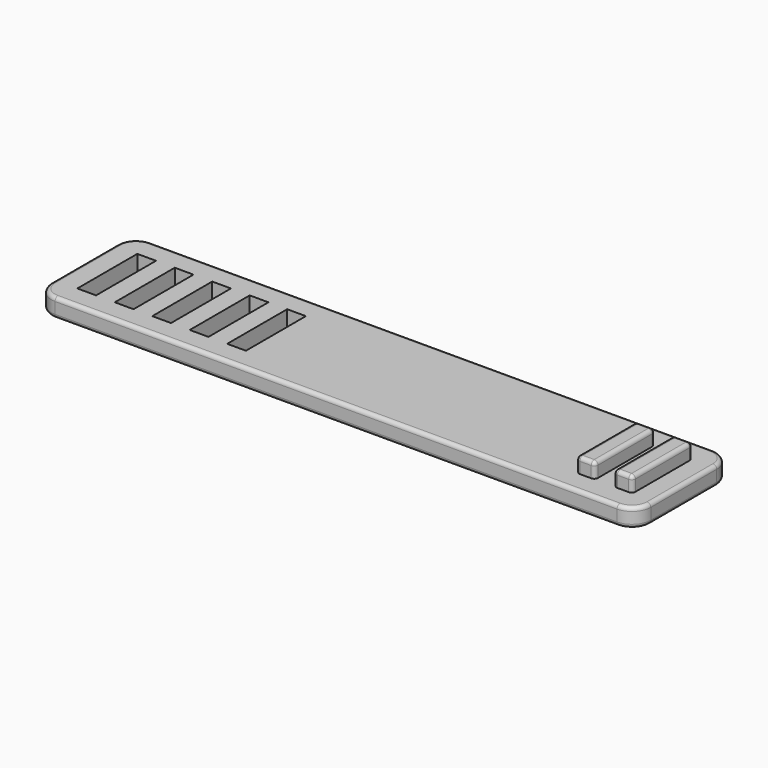
from build123d import *

# Parameters (mm, degrees)
F0_W     = 6.35
F0_H     = 25.4
F0_R     = 17.5576306553
F1_DEPTH = 6.35
F2_R     = 1.27
F3_W     = 6.35
F3_H     = 25.4
F4_DEPTH = 5.08
F5_R     = 1.27


# Not quite as in the source:
# - a feature names something its author has since deleted; it is built from what else it names


with BuildPart() as f1:
    # F0 (on Top) → F1 (new body)
    with BuildSketch(Plane.XY):
        with BuildLine():
            ThreePointArc((101.6, 13.97), (99.7401280605, 18.4601280605), (95.25, 20.32))
            Line((95.25, 20.32), (-95.25, 20.32))
            ThreePointArc((-95.25, 20.32), (-99.7401280605, 18.4601280605), (-101.6, 13.97))
            Line((-101.6, 13.97), (-101.6, -13.97))
            ThreePointArc((-101.6, -13.97), (-99.7401280605, -18.4601280605), (-95.25, -20.32))
            Line((-95.25, -20.32), (95.25, -20.32))
            ThreePointArc((95.25, -20.32), (99.7401280605, -18.4601280605), (101.6, -13.97))
            Line((101.6, -13.97), (101.6, 13.97))
        make_face()
        with Locations((-90.6151607633, 0)):
            Rectangle(F0_W, F0_H, mode=Mode.SUBTRACT)
        with Locations((-77.9151607633, 0)):
            Rectangle(F0_W, F0_H, mode=Mode.SUBTRACT)
        with Locations((-65.2151607633, 0)):
            Rectangle(F0_W, F0_H, mode=Mode.SUBTRACT)
        with Locations((-52.5151607633, 0)):
            Rectangle(F0_W, F0_H, mode=Mode.SUBTRACT)
        with Locations((-39.8151607633, 0)):
            Rectangle(F0_W, F0_H, mode=Mode.SUBTRACT)
        with Locations((4.1378471069, 0)):
            Circle(F0_R, mode=Mode.SUBTRACT)
        with Locations((4.1378471069, 0)):
            Circle(F0_R)
    extrude(amount=F1_DEPTH)

    # F2
    f2_edges = [f1.edges().sort_by_distance(p)[0] for p in [
        (0, -20.32, 0),
        (0, -20.32, 6.35),
    ]]
    fillet(f2_edges, radius=F2_R)

    # F3 (on face) → F4 (join)
    with BuildSketch(Plane.XY.offset(6.35)):
        with Locations((78.503764081, 0)):
            Rectangle(F3_W, F3_H)
        with Locations((91.203764081, 0)):
            Rectangle(F3_W, F3_H)
    extrude(amount=F4_DEPTH)

    # F5
    f5_edges = [f1.edges().sort_by_distance(p)[0] for p in [
        (81.678764, 0, 11.43),
        (78.503764, -12.7, 11.43),
        (75.328764, 0, 11.43),
        (78.503764, 12.7, 11.43),
        (88.028764, 0, 11.43),
        (94.378764, 0, 11.43),
        (91.203764, -12.7, 11.43),
        (91.203764, 12.7, 11.43),
        (94.378764, -12.7, 8.89),
        (88.028764, -12.7, 8.89),
        (81.678764, -12.7, 8.89),
        (75.328764, -12.7, 8.89),
        (81.678764, 12.7, 8.89),
        (94.378764, 12.7, 8.89),
        (88.028764, 12.7, 8.89),
        (75.328764, 12.7, 8.89),
    ]]
    fillet(f5_edges, radius=F5_R)


solid = f1.part
